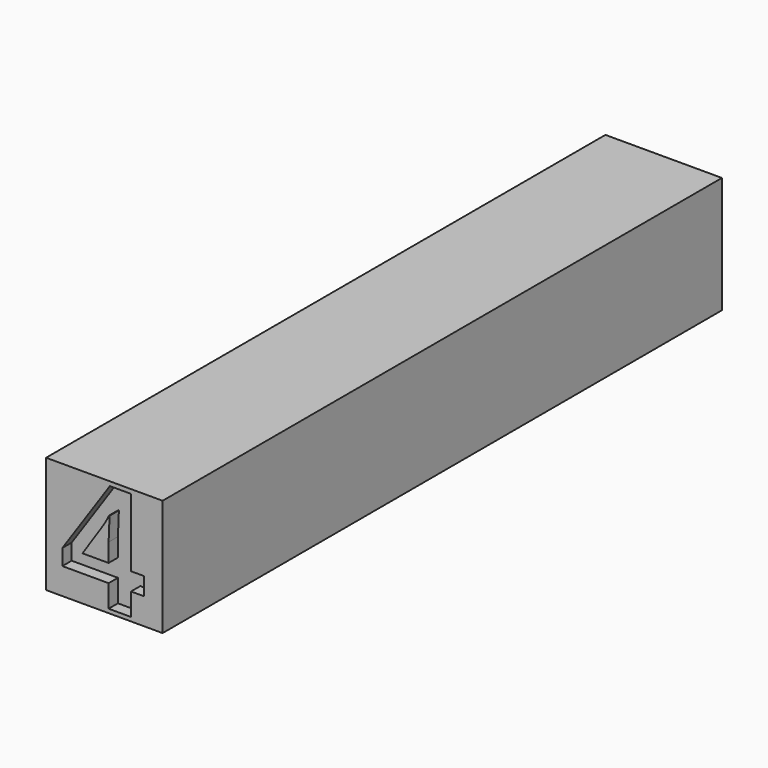
from build123d import *

# Parameters (mm, degrees)
F0_W         = 25.4
F0_H         = 25.4
F1_DEPTH     = 152.4
F2_TEXT_SIZE = 33.0896607516
F3_DEPTH     = 2.54


# Not quite as in the source:
# - Text() gives the source's letters only with a copy of the font that has no kerning and outlines rounded to 1/6400 em; it was checked with that copy


with BuildPart() as f1:
    # F0 (on Front) → F1 (new body)
    with BuildSketch(Plane.XZ):
        with Locations((12.7, 12.7)):
            Rectangle(F0_W, F0_H)
    extrude(amount=F1_DEPTH)

    # F2 (on face) → F3 (cut)
    with BuildSketch(Plane.XZ.offset(152.4)):
        with Locations((2.9820885975, 0.8600634173)):
            Text('4', F2_TEXT_SIZE, font='Open Sans', font_style=FontStyle.BOLD, text_align=(TextAlign.LEFT, TextAlign.BOTTOM))
    extrude(amount=-F3_DEPTH, mode=Mode.SUBTRACT)


solid = f1.part
